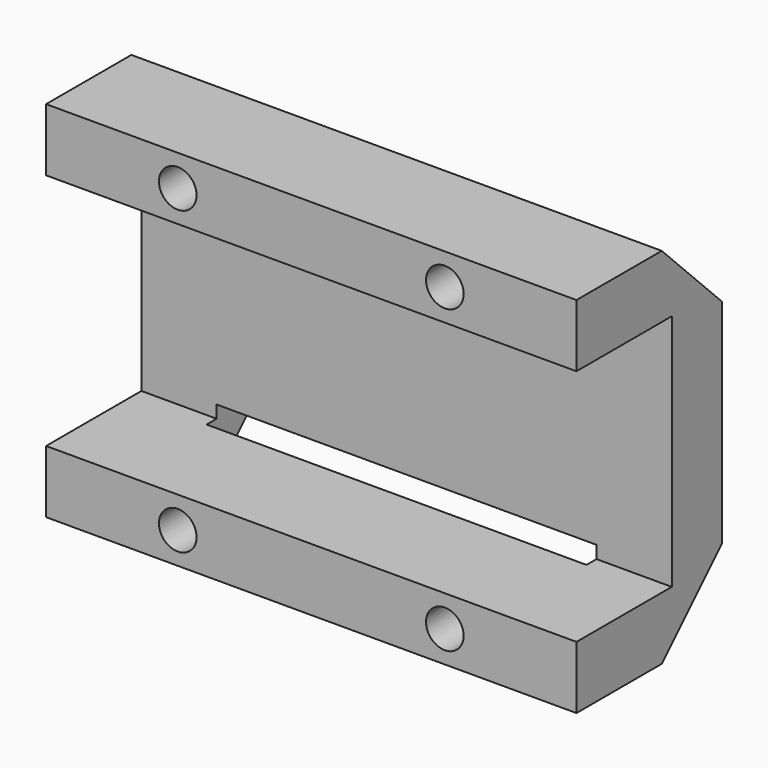
from build123d import *

# Parameters (mm, degrees)
F1_DEPTH = 42.3
F2_W     = 30.3
F2_H     = 6
F3_DEPTH = 6
F4_SIZE  = 6
F5_R     = 1.5
F6_DEPTH = 8.501
F7_R     = 1.5
F8_DEPTH = 8.501


# Not quite as in the source:
# - a feature names something its author has since deleted; it is built from what else it names


with BuildPart() as f1:
    # F0 (on Right) → F1 (new body)
    with BuildSketch(Plane.YZ):
        Polygon((0, 9.5), (9.5, 9.5), (9.5, -9.5), (0, -9.5), (0, -14.5), (14.5, -14.5), (14.5, 14.5), (0, 14.5), align=None)
    extrude(amount=F1_DEPTH)

    # F2 (on face) → F3 (cut)
    with BuildSketch(Plane(origin=(0, 14.5, 0), x_dir=(-1, 0, 0), z_dir=(0, 1, 0))):
        with Locations((-21.15, 11.5)):
            Rectangle(F2_W, F2_H)
        with Locations((-21.15, -11.5)):
            Rectangle(F2_W, F2_H)
    extrude(amount=-F3_DEPTH, mode=Mode.SUBTRACT)

    # F4
    f4_edges = [f1.edges().sort_by_distance(p)[0] for p in [
        (3, 14.5, -14.5),
        (39.3, 14.5, -14.5),
        (39.3, 14.5, 14.5),
        (3, 14.5, 14.5),
    ]]
    chamfer(f4_edges, length=F4_SIZE)

    # F5 (on face) → F6 (cut, through all)
    with BuildSketch(Plane(origin=(0, 8.5, 0), x_dir=(-1, 0, 0), z_dir=(0, 1, 0))):
        with Locations((-31.8, 12)):
            Circle(F5_R)
        with Locations((-10.5, 12)):
            Circle(F5_R)
    extrude(amount=-F6_DEPTH, mode=Mode.SUBTRACT)

    # F7 (on face) → F8 (cut, through all)
    with BuildSketch(Plane(origin=(0, 8.5, 0), x_dir=(-1, 0, 0), z_dir=(0, 1, 0))):
        with Locations((-31.8, -12)):
            Circle(F7_R)
        with Locations((-10.5, -12)):
            Circle(F7_R)
    extrude(amount=-F8_DEPTH, mode=Mode.SUBTRACT)


solid = f1.part
